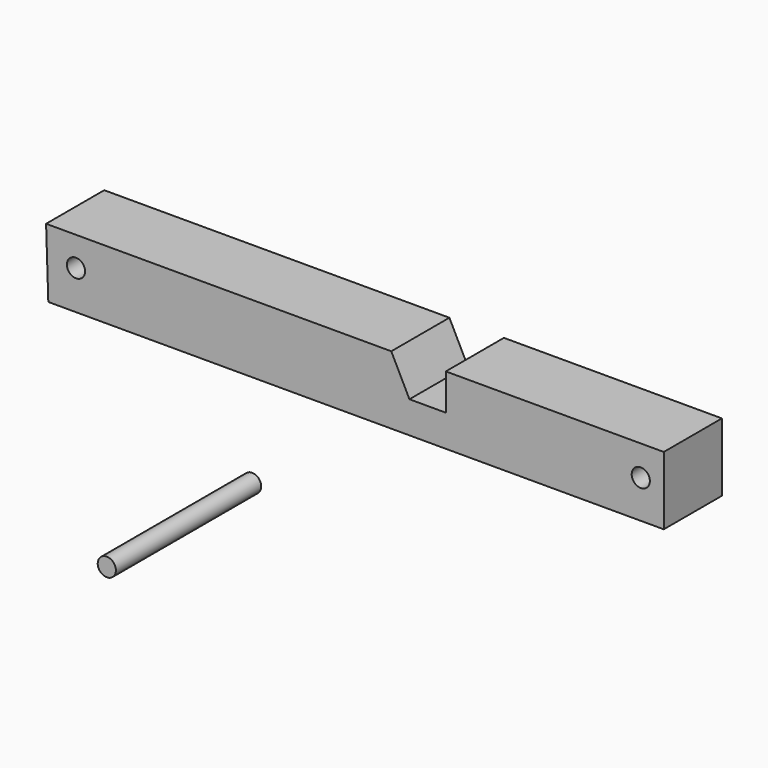
from build123d import *

# Parameters (mm, degrees)
F1_DEPTH = 25.4
F2_R     = 3.175
F3_DEPTH = 25.401
F4_R     = 3.175
F5_DEPTH = 63.5


# Not quite as in the source:
# - a feature names something its author has since deleted; it is built from what else it names


with BuildPart() as f1:
    # F0 (on Front) → F1 (new body)
    with BuildSketch(Plane.XZ):
        Polygon((132.3305627346, 43.7965765595), (-83.5694372654, 43.7965765595), (-82.7916205839, 19.9840765595), (132.3305627346, 19.9840765595), align=None)
    extrude(amount=F1_DEPTH)

    # F2 (on face) → F3 (cut, through all)
    with BuildSketch(Plane.XZ.offset(25.4)):
        with Locations((-73.1171146035, 33.582534641)):
            Circle(F2_R)
        Polygon((43.4305627346, 31.0965765595), (56.1305627346, 31.0965765595), (56.1305627346, 43.7965765595), (37.0805627346, 43.7965765595), align=None)
        with Locations((124.286480248, 33.2658700645)):
            Circle(F2_R)
    extrude(amount=-F3_DEPTH, mode=Mode.SUBTRACT)


with BuildPart() as f5:
    # F4 (on Front) → F5 (new body)
    with BuildSketch(Plane.XZ):
        with Locations((-31.8689309061, -29.5055080205)):
            Circle(F4_R)
    extrude(amount=F5_DEPTH)


solid = Compound([f1.part, f5.part])
